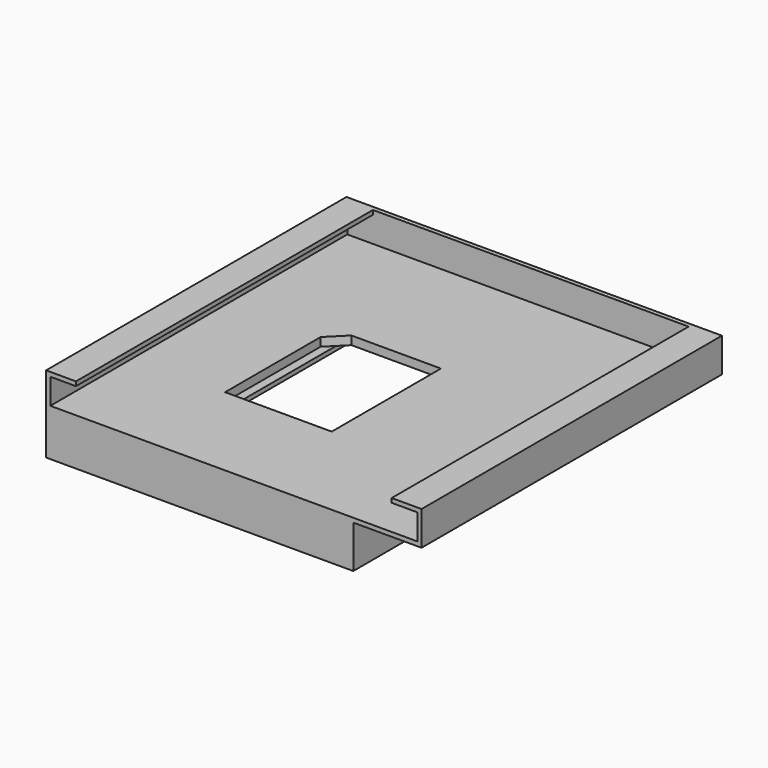
from build123d import *

# Parameters (mm, degrees)
F1_DEPTH = 88
F3_DEPTH = 1
F4_DEPTH = 88
F6_DEPTH = 1
F8_DEPTH = 2


with BuildPart() as f1:
    # F0 (on Front) → F1 (new body)
    with BuildSketch(Plane.XZ):
        Polygon((43, 0), (0, 0), (-43, 0), (-43, 6), (-37, 6), (-37, 7), (-44, 7), (-44, -1), (0, -1), (28, -1), (44, -1), (44, 7), (37, 7), (37, 6), (43, 6), align=None)
    extrude(amount=F1_DEPTH)

    # F2 (on face) → F3 (join)
    with BuildSketch(Plane(origin=(0, 0, 0), x_dir=(-1, 0, 0), z_dir=(0, 1, 0))):
        Polygon((37, 7), (-37, 7), (-37, 6), (-43, 6), (-43, 0), (43, 0), (43, 6), (37, 6), align=None)
    extrude(amount=-F3_DEPTH)

    # F0 (on Front) → F4 (join)
    with BuildSketch(Plane.XZ):
        Polygon((0, -1), (-44, -1), (-44, -11), (-29, -11), (-29, -10), (-43, -10), (-43, -2), (0, -2), (27, -2), (27, -10), (13, -10), (13, -11), (28, -11), (28, -2), (28, -1), align=None)
    extrude(amount=F4_DEPTH)

    # F5 (on face) → F6 (join)
    with BuildSketch(Plane.XZ.offset(88)):
        Polygon((-29, -10), (-29, -11), (13, -11), (13, -10), (27, -10), (27, -2), (-43, -2), (-43, -10), align=None)
    extrude(amount=-F6_DEPTH)

    # F7 (on Top) → F8 (cut)
    with BuildSketch(Plane.XY):
        Polygon((-21.4086160213, -63.8053458929), (3.5913839787, -63.8053458929), (3.5913839787, -31.8053458929), (-17.4086160213, -31.8053458929), (-21.4086160213, -35.8053458929), align=None)
    extrude(amount=-F8_DEPTH, mode=Mode.SUBTRACT)


solid = f1.part
